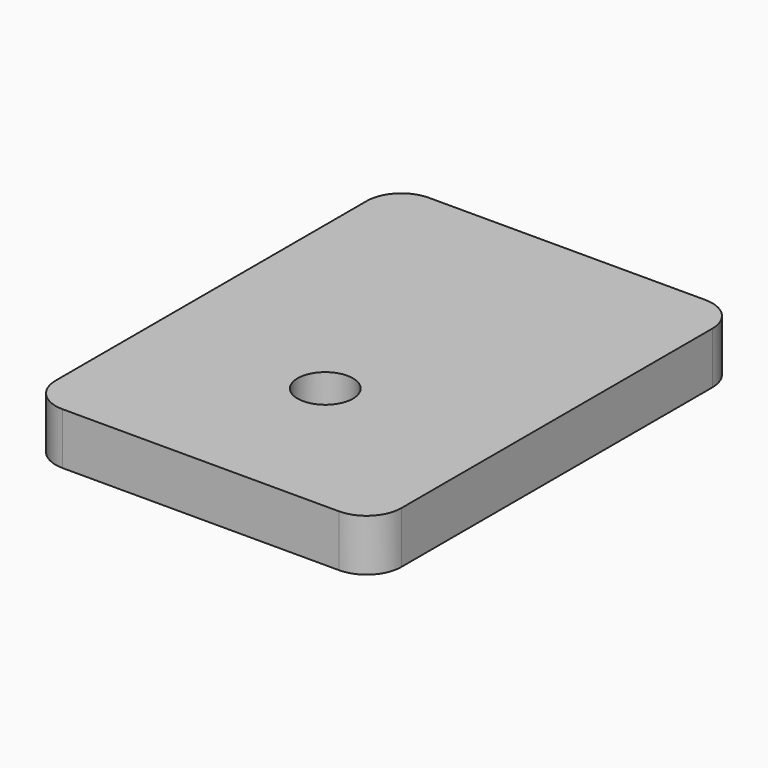
from build123d import *

# Parameters (mm, degrees)
F0_R     = 1.6
F1_DEPTH = 3


# Not quite as in the source:
# - ends of sketch curves that miss each other by under 0.0002 mm in the source are joined


with BuildPart() as f1:
    # F0 (on Top) → F1 (new body)
    with BuildSketch(Plane.XY):
        with BuildLine():
            Line((8.000003, 13.251824), (-7.999997, 13.251824))
            ThreePointArc((-7.999997, 13.251824), (-9.4142105624, 12.6660375624), (-9.999997, 11.251824))
            Line((-9.999997, 11.251824), (-10.000002, -11.251824))
            ThreePointArc((-10.000002, -11.251824), (-9.4142155624, -12.6660375624), (-8.000002, -13.251824))
            Line((-8.000002, -13.251824), (7.999998, -13.251824))
            ThreePointArc((7.999998, -13.251824), (9.4142115624, -12.6660375624), (9.999998, -11.251824))
            Line((9.999998, -11.251824), (9.999988, 11.251824))
            ThreePointArc((9.999988, 11.251824), (9.4142165624, 12.6660375624), (8.000003, 13.251824))
        make_face()
        with Locations((-1.2e-05, -4.248124)):
            Circle(F0_R, mode=Mode.SUBTRACT)
    extrude(amount=F1_DEPTH)


solid = f1.part
